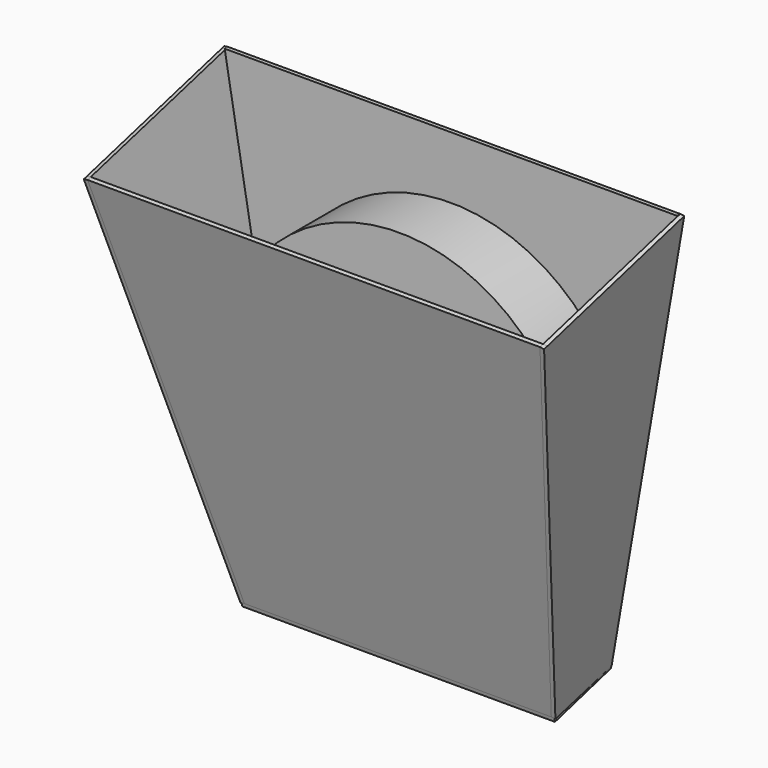
from build123d import *

# Parameters (mm, degrees)
F2_DEPTH  = 3.175
F3_R      = 139.7
F4_DEPTH  = 50.8
F8_DEPTH  = 3.175
F10_DEPTH = 3.175
F12_W     = 245.7978874445
F12_H     = 57.0418144985
F13_DEPTH = 3.175


with BuildPart() as f2:
    # F1 (on Front) → F2 (new body)
    with BuildSketch(Plane.XZ):
        Polygon((120.65, 266.7), (177.8, 596.9), (-177.8, 596.9), (-120.65, 266.7), align=None)
    extrude(amount=-F2_DEPTH)


with BuildPart() as f4:
    # F3 (on face) → F4 (new body)
    with BuildSketch(Plane.XZ):
        with Locations((0, 408.4407389164)):
            Circle(F3_R)
    extrude(amount=F4_DEPTH)


with BuildPart() as f8:
    # F7 (on face) → F8 (new body)
    with BuildSketch(Plane(origin=(0, 14.539153526, 3.8957544459), x_dir=(-1, 0, 0), z_dir=(0, 0.9659258263, 0.2588190451))):
        Polygon((120.65, 257.6124178713), (177.8, 576.5611257119), (-177.8, 576.5611257119), (-120.65, 257.6124178713), align=None)
    extrude(amount=F8_DEPTH)


with BuildPart() as f10:
    # F9 (on face) → F10 (new body)
    with BuildSketch(Plane(origin=(-72.1731684636, 3.347089997, -12.4915099264), x_dir=(-0.0449800713, -0.99895755, -0.0077850123), z_dir=(-0.9843233273, 0.0456488032, -0.1703636528))):
        Polygon((135.102368204, 583.7099916129), (0.1788925906, 618.477983858), (0.1788925906, 283.3688038882), (52.4708201773, 270.4134080558), align=None)
        Polygon((138.1769790582, 582.9177051272), (135.102368204, 583.7099916129), (52.4708201773, 270.4134080558), (55.5408350126, 269.6036958163), align=None)
    extrude(amount=F10_DEPTH)


with BuildPart() as f11_1:
    # F11: instance of F10
    add(f10.part.mirror(Plane.YZ))


with BuildPart() as f13:
    # F12 (on face) → F13 (new body)
    with BuildSketch(Plane(origin=(0, -66.675, 248.8344875947), x_dir=(1, 0, 0), z_dir=(0, 0.2588190451, -0.9659258263))):
        with Locations((0, -43.5729465781)):
            Rectangle(F12_W, F12_H)
    extrude(amount=F13_DEPTH)


solid = Compound([f2.part, f4.part, f8.part, f10.part, f11_1.part, f13.part])
